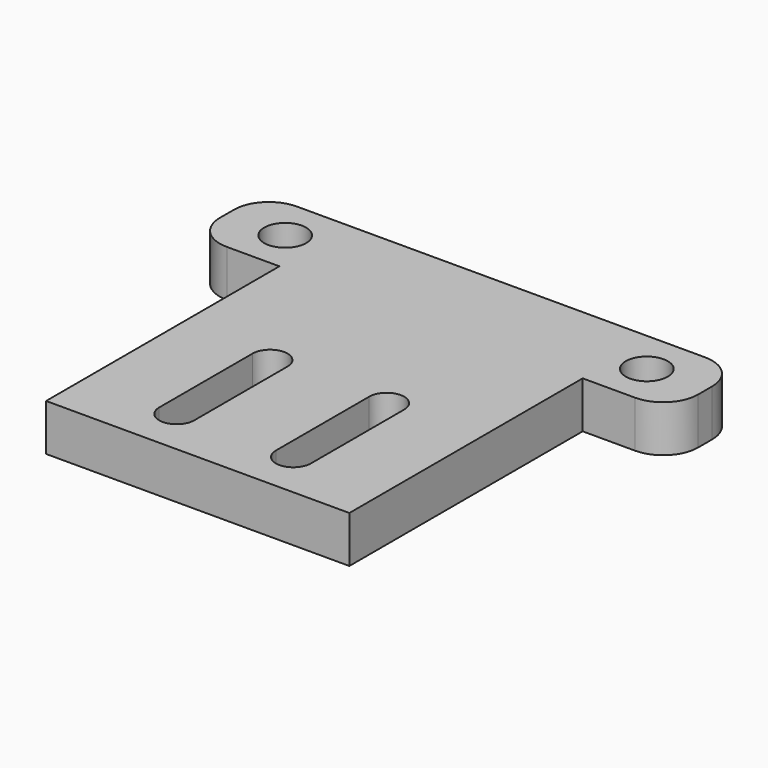
from build123d import *

# Parameters (mm, degrees)
F0_R     = 1.8
F0_W     = 26
F0_H     = 25
F1_DEPTH = 4
F2_R     = 3


# Not quite as in the source:
# - a feature names something its author has since deleted; it is built from what else it names


with BuildPart() as f1:
    # F0 (on Top) → F1 (new body)
    with BuildSketch(Plane.XY):
        Polygon((0, 7.5), (-41, 7.5), (-41, 0), (-33.5, 0), (-7.5, 0), (0, 0), align=None)
        with Locations((-36, 3.75)):
            Circle(F0_R, mode=Mode.SUBTRACT)
        with Locations((-5, 3.75)):
            Circle(F0_R, mode=Mode.SUBTRACT)
        with Locations((-20.5, -12.5)):
            Rectangle(F0_W, F0_H)
        with BuildLine():
            Line((-27, -21), (-27, -11))
            ThreePointArc((-27, -11), (-25.5, -9.5), (-24, -11))
            Line((-24, -11), (-24, -21))
            ThreePointArc((-24, -21), (-25.5, -22.5), (-27, -21))
        make_face(mode=Mode.SUBTRACT)
        with BuildLine():
            Line((-17, -21), (-17, -11))
            ThreePointArc((-17, -11), (-15.5, -9.5), (-14, -11))
            Line((-14, -11), (-14, -21))
            ThreePointArc((-14, -21), (-15.5, -22.5), (-17, -21))
        make_face(mode=Mode.SUBTRACT)
    extrude(amount=F1_DEPTH)

    # F2
    f2_edges = [f1.edges().sort_by_distance(p)[0] for p in [
        (0, 0, 2),
        (0, 7.5, 2),
        (-41, 0, 2),
        (-41, 7.5, 2),
    ]]
    fillet(f2_edges, radius=F2_R)


solid = f1.part
